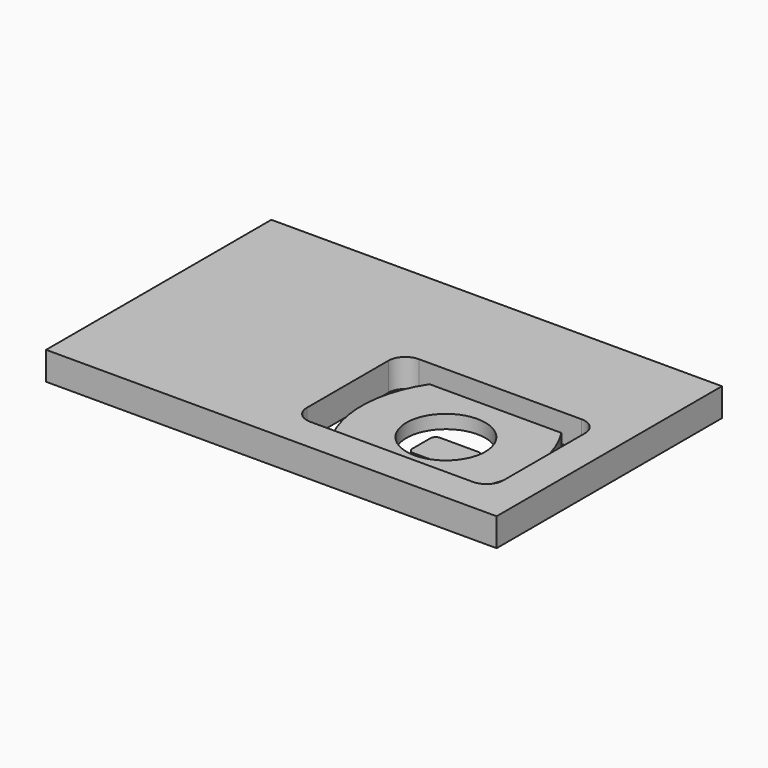
from build123d import *

# Parameters (mm, degrees)
F1_W     = 400
F1_H     = 250
F1_W_2   = 174.5
F1_H_2   = 120.5
F2_DEPTH = 25
F1_R     = 35
F3_DEPTH = 12
F1_W_3   = 43.5
F1_H_3   = 29.5
F4_DEPTH = 1
F5_R     = 4.75
F6_R     = 15


# Not quite as in the source:
# - a feature names something its author has since deleted; it is built from what else it names


with BuildPart() as f2:
    # F1 (on Top) → F2 (new body)
    with BuildSketch(Plane.XY):
        with Locations((-82.75, 34.75)):
            Rectangle(F1_W, F1_H)
        Rectangle(F1_W_2, F1_H_2, mode=Mode.SUBTRACT)
    extrude(amount=F2_DEPTH)

    # F6
    f6_edges = [f2.edges().sort_by_distance(p)[0] for p in [
        (87.25, -60.25, 12.5),
        (87.25, 60.25, 12.5),
        (-87.25, 60.25, 12.5),
        (-87.25, -60.25, 12.5),
    ]]
    fillet(f6_edges, radius=F6_R)


with BuildPart() as f3:
    # F1 (on Top) → F3 (new body)
    with BuildSketch(Plane.XY):
        with BuildLine():
            Line((58.5164654425, 55), (-58.5164654425, 55))
            ThreePointArc((-58.5164654425, 55), (-75, 0), (-58.5164654425, -55))
            Line((-58.5164654425, -55), (58.5164654425, -55))
            ThreePointArc((58.5164654425, -55), (75, 0), (58.5164654425, 55))
        make_face()
        Circle(F1_R, mode=Mode.SUBTRACT)
    extrude(amount=F3_DEPTH)


with BuildPart() as f4:
    # F1 (on Top) → F4 (new body)
    with BuildSketch(Plane.XY):
        Rectangle(F1_W_3, F1_H_3)
    extrude(amount=-F4_DEPTH)

    # F5
    f5_edges = [f4.edges().sort_by_distance(p)[0] for p in [
        (21.75, -14.75, -0.5),
        (21.75, 14.75, -0.5),
        (-21.75, -14.75, -0.5),
        (-21.75, 14.75, -0.5),
    ]]
    fillet(f5_edges, radius=F5_R)


solid = Compound([f2.part, f3.part, f4.part])
